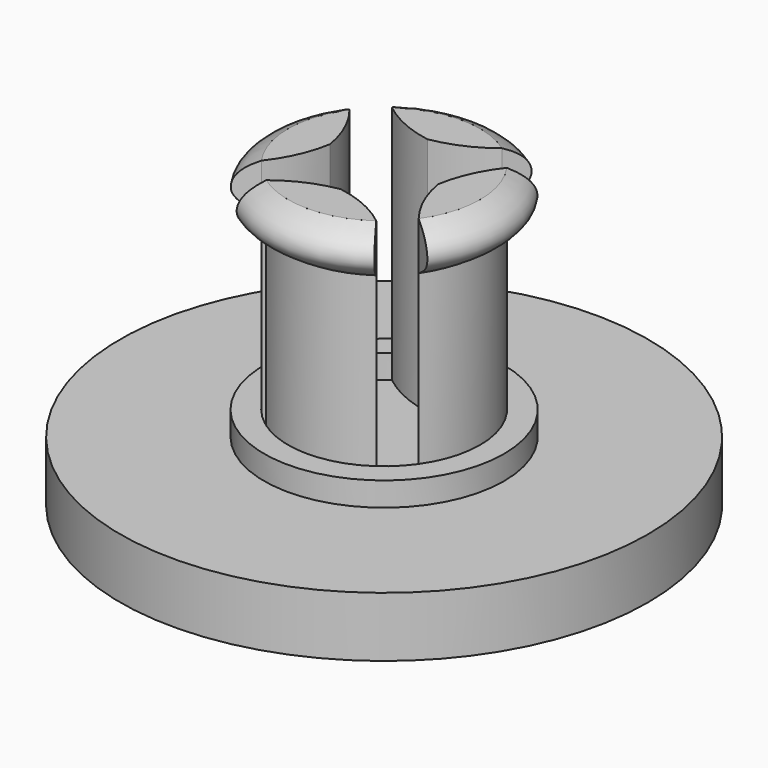
from build123d import *

# Parameters (mm, degrees)
F0_R          = 11
F0_R_2        = 4
F0_R_3        = 3.8
F1_DEPTH      = 2.5
F3_ANGLE_BACK = 35
F3_ANGLE      = 70
F4_T1_DEPTH   = 18.8347389731
F5_COUNT      = 4
F7_R          = 5
F7_R_2        = 4
F8_DEPTH      = 1


# Not quite as in the source:
# - a fillet or chamfer that OpenCascade refuses, or shapes differently, is made with other operations: its cross-section is extruded or revolved along the edge and cut away or added


with BuildPart() as f1:
    # F0 (on Top) → F1 (new body)
    with BuildSketch(Plane.XY):
        Circle(F0_R)
        Circle(F0_R_2, mode=Mode.SUBTRACT)
        Circle(F0_R_2)
        Circle(F0_R_3, mode=Mode.SUBTRACT)
        Circle(F0_R_3)
    extrude(amount=F1_DEPTH)


with BuildPart() as f3:
    # F2 (on Right) → F3 (revolve)
    with BuildSketch(Plane.YZ, mode=Mode.PRIVATE) as f3_sk:
        Polygon((2.2330522054, 12.5), (2.2330522054, 2.5), (4, 2.5), (4, 10.5), (4, 12.5), align=None)
        with BuildLine():
            add(Edge.make_bspline(
                [(4, 12.5), (4.8024506061, 12.181599044), (5.20459018, 11.4267656029), (4.7883662135, 10.9662323332), (4, 10.5)],
                knots=[0, 0, 0, 0, 0.4999497915, 1, 1, 1, 1], degree=3))
            Line((4, 12.5), (4, 10.5))
        make_face()
    revolve(f3_sk.sketch.rotate(Axis((0, 0, 5.986657925), (0, 0, 1)), -F3_ANGLE_BACK), axis=Axis((0, 0, 5.986657925), (0, 0, 1)), revolution_arc=F3_ANGLE)

    # F4: fillet of radius 5 on 2 edges, made by hand

    # F4_s2 → F4_t1 (cut)
    with BuildSketch(Plane.XY.offset(-1.9173694866)):
        with BuildLine():
            ThreePointArc((0.2539943419, 2.2185601246), (-1.0945850785, 2.5683216052), (-2.2943057454, 3.2766081772))
            Line((-2.2943057454, 3.2766081772), (-1.2808261261, 1.829209279))
            ThreePointArc((-1.2808261261, 1.829209279), (-0.5490850558, 2.1644924933), (0.2539943419, 2.2185601246))
        make_face()
        with BuildLine():
            ThreePointArc((-0.2539943419, 2.2185601246), (1.0945850785, 2.5683216052), (2.2943057454, 3.2766081772))
            Line((2.2943057454, 3.2766081772), (1.2808261261, 1.829209279))
            ThreePointArc((1.2808261261, 1.829209279), (0.5490850558, 2.1644924933), (-0.2539943419, 2.2185601246))
        make_face()
    extrude(amount=F4_T1_DEPTH, mode=Mode.SUBTRACT)


with BuildPart() as f5_1:
    # F5: instance of F3
    add(f3.part.rotate(Axis((0, 0, 5.986657925), (0, 0, 1)), 1 * 360 / F5_COUNT))


with BuildPart() as f5_2:
    # F5: instance of F3
    add(f3.part.rotate(Axis((0, 0, 5.986657925), (0, 0, 1)), 2 * 360 / F5_COUNT))


with BuildPart() as f5_3:
    # F5: instance of F3
    add(f3.part.rotate(Axis((0, 0, 5.986657925), (0, 0, 1)), 3 * 360 / F5_COUNT))


with BuildPart() as f6_1:
    # F6: copy of F1
    add(f1.part)


with BuildPart() as f8:
    # F7 (on face) → F8 (new body)
    with BuildSketch(Plane.XY.offset(2.5)):
        Circle(F7_R)
        Circle(F7_R_2, mode=Mode.SUBTRACT)
    extrude(amount=F8_DEPTH)


solid = Compound([f1.part, f3.part, f5_1.part, f5_2.part, f5_3.part, f6_1.part, f8.part])
